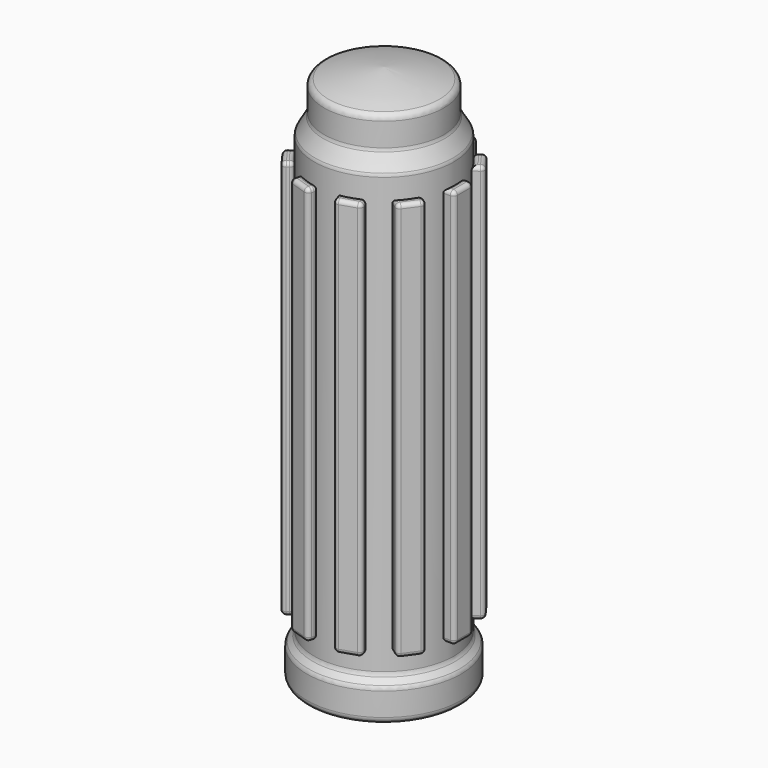
from build123d import *

# Parameters (mm, degrees)
F2_R     = 1.6
F4_W     = 6
F4_H     = 100
F6_R     = 1
F7_COUNT = 10


with BuildPart() as f1:
    # F0 (on Front) → F1 (revolve)
    with BuildSketch(Plane.XZ):
        with BuildLine():
            Line((10.75, 127), (10.75, 0))
            Line((10.75, 0), (19.325, 0))
            Line((19.325, 0), (19.325, 8))
            Line((19.325, 8), (17.5, 10.1749503065))
            Line((17.5, 10.1749503065), (17.5, 120.1749503065))
            Line((17.5, 120.1749503065), (15, 124.5050773254))
            Line((15, 124.5050773254), (15, 132.0050773254))
            ThreePointArc((15, 132.0050773254), (7.584478537, 133.9256474347), (0, 135))
            Line((0, 135), (0, 127))
            Line((0, 127), (10.75, 127))
        make_face()
    revolve(axis=Axis((0, 0, 77.9052749614), (0, 0, 1)))

    # F2
    f2_edges = [f1.edges().sort_by_distance(p)[0] for p in [
        (-15, 0, 132.005077),
        (-17.5, 0, 120.17495),
        (-15, 0, 124.505077),
        (-17.5, 0, 10.17495),
        (-19.325, 0, 8),
        (-19.325, 0, 0),
    ]]
    fillet(f2_edges, radius=F2_R)


with BuildPart() as f5:
    # F4 (on offset) → F5 (new body, up to the next surface of F1)
    with BuildSketch(Plane.YZ.offset(20)):
        with Locations((0, 65)):
            Rectangle(F4_W, F4_H)
    extrude(until=Until.NEXT, target=f1.part, dir=(-1, 0, 0))

    # F6
    f6_edges = [f5.edges().sort_by_distance(p)[0] for p in [
        (20, 0, 115),
        (20, -3, 65),
        (20, 0, 15),
        (20, 3, 65),
        (17.24094, 3, 65),
        (18.62047, -3, 115),
        (17.435115, -1.505582, 115),
        (17.435115, 1.505582, 115),
        (18.62047, 3, 115),
        (18.62047, 3, 15),
        (17.435115, 1.505582, 15),
        (17.435115, -1.505582, 15),
        (18.62047, -3, 15),
    ]]
    fillet(f6_edges, radius=F6_R)


with BuildPart() as f7_1:
    # F7: instance of F5
    add(f5.part.rotate(Axis((0, 0, 0), (0, 0, 1)), 1 * 360 / F7_COUNT))


with BuildPart() as f7_2:
    # F7: instance of F5
    add(f5.part.rotate(Axis((0, 0, 0), (0, 0, 1)), 2 * 360 / F7_COUNT))


with BuildPart() as f7_3:
    # F7: instance of F5
    add(f5.part.rotate(Axis((0, 0, 0), (0, 0, 1)), 3 * 360 / F7_COUNT))


with BuildPart() as f7_4:
    # F7: instance of F5
    add(f5.part.rotate(Axis((0, 0, 0), (0, 0, 1)), 4 * 360 / F7_COUNT))


with BuildPart() as f7_5:
    # F7: instance of F5
    add(f5.part.rotate(Axis((0, 0, 0), (0, 0, 1)), 5 * 360 / F7_COUNT))


with BuildPart() as f7_6:
    # F7: instance of F5
    add(f5.part.rotate(Axis((0, 0, 0), (0, 0, 1)), 6 * 360 / F7_COUNT))


with BuildPart() as f7_7:
    # F7: instance of F5
    add(f5.part.rotate(Axis((0, 0, 0), (0, 0, 1)), 7 * 360 / F7_COUNT))


with BuildPart() as f7_8:
    # F7: instance of F5
    add(f5.part.rotate(Axis((0, 0, 0), (0, 0, 1)), 8 * 360 / F7_COUNT))


with BuildPart() as f7_9:
    # F7: instance of F5
    add(f5.part.rotate(Axis((0, 0, 0), (0, 0, 1)), 9 * 360 / F7_COUNT))


solid = Compound([f1.part, f5.part, f7_1.part, f7_2.part, f7_3.part, f7_4.part, f7_5.part, f7_6.part, f7_7.part, f7_8.part, f7_9.part])
